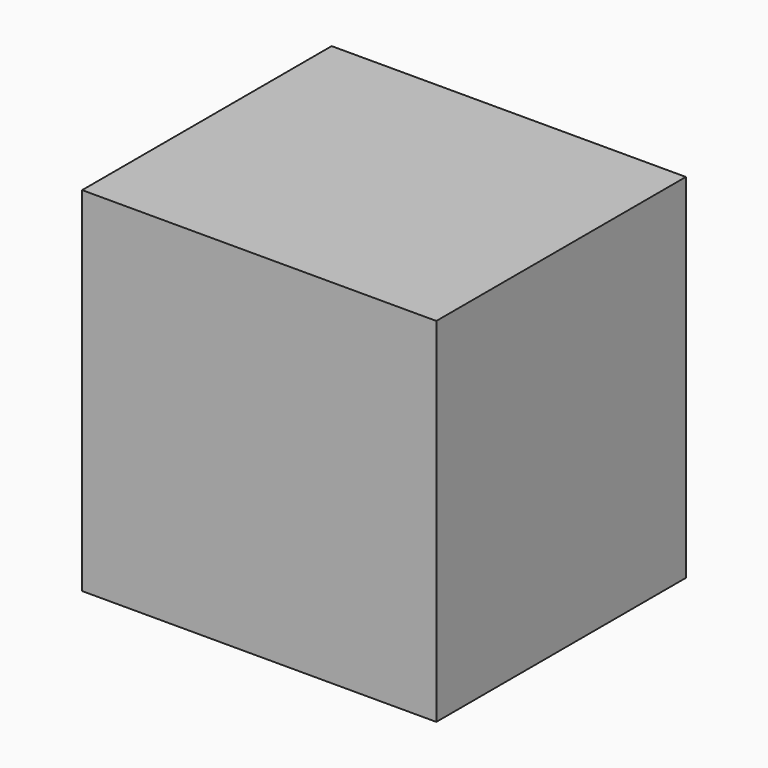
from build123d import *

# Parameters (mm, degrees)
F0_W     = 74.422
F0_H     = 74.168
F1_DEPTH = 65.532


# Not quite as in the source:
# - the program builds the solid bodies; features that only make, move or delete a surface that nothing else refers to are left out


with BuildPart() as f1:
    # F0 (on Front) → F1 (new body)
    with BuildSketch(Plane.XZ):
        with Locations((12.2112619318, -10.9315998852)):
            Rectangle(F0_W, F0_H)
    extrude(amount=F1_DEPTH)


solid = f1.part
